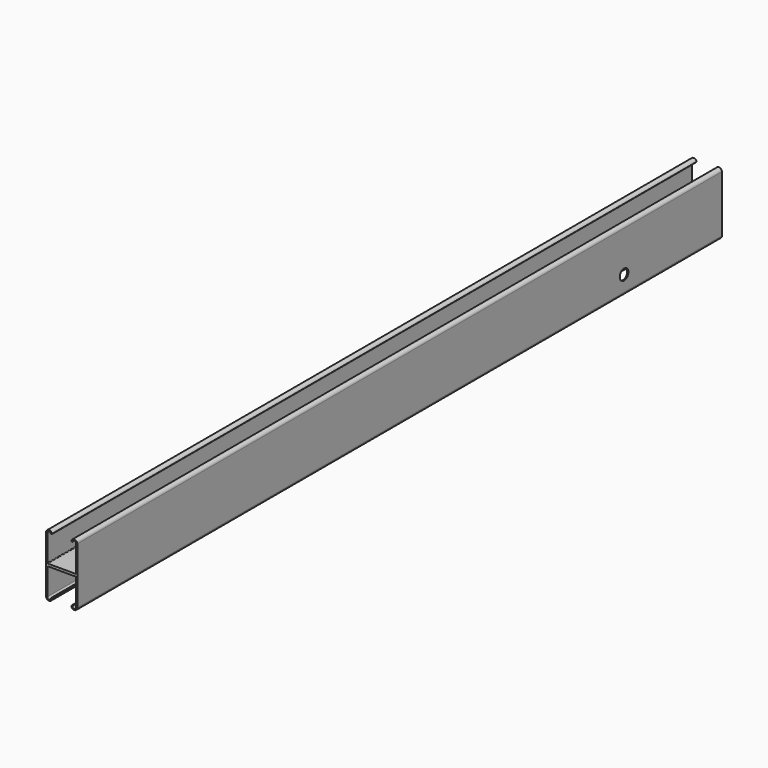
from build123d import *

# Parameters (mm, degrees)
F1_DEPTH = 533.4
F2_R     = 0.79374
F3_R     = 7.14375
F4_DEPTH = 41.276


# Not quite as in the source:
# - a fillet or chamfer is up to 0.001 mm smaller than in the source, because OpenCascade refuses the exact size


with BuildPart() as f1:
    # F0 (on Front) → F1 (new body, symmetric)
    with BuildSketch(Plane.XZ):
        with BuildLine():
            Line((0, 37.30625), (0, 0))
            Line((0, 0), (20.6375, 0))
            Line((20.6375, 0), (20.6375, 1.5875))
            Line((20.6375, 1.5875), (1.5875, 1.5875))
            Line((1.5875, 1.5875), (1.5875, 37.30625))
            ThreePointArc((1.5875, 37.30625), (3.96875, 39.6875), (6.35, 37.30625))
            Line((6.35, 37.30625), (7.9375, 37.30625))
            ThreePointArc((7.9375, 37.30625), (3.96875, 41.275), (0, 37.30625))
        make_face()
        with BuildLine():
            Line((20.6375, 0), (0, 0))
            Line((0, 0), (0, -37.30625))
            ThreePointArc((0, -37.30625), (3.96875, -41.275), (7.9375, -37.30625))
            Line((7.9375, -37.30625), (6.35, -37.30625))
            ThreePointArc((6.35, -37.30625), (3.96875, -39.6875), (1.5875, -37.30625))
            Line((1.5875, -37.30625), (1.5875, -1.5875))
            Line((1.5875, -1.5875), (20.6375, -1.5875))
            Line((20.6375, -1.5875), (20.6375, 0))
        make_face()
        with BuildLine():
            Line((20.6375, 1.5875), (20.6375, 0))
            Line((20.6375, 0), (41.275, 0))
            Line((41.275, 0), (41.275, 37.30625))
            ThreePointArc((41.275, 37.30625), (37.30625, 41.275), (33.3375, 37.30625))
            Line((33.3375, 37.30625), (34.925, 37.30625))
            ThreePointArc((34.925, 37.30625), (37.30625, 39.6875), (39.6875, 37.30625))
            Line((39.6875, 37.30625), (39.6875, 1.5875))
            Line((39.6875, 1.5875), (20.6375, 1.5875))
        make_face()
        with BuildLine():
            Line((41.275, 0), (20.6375, 0))
            Line((20.6375, 0), (20.6375, -1.5875))
            Line((20.6375, -1.5875), (39.6875, -1.5875))
            Line((39.6875, -1.5875), (39.6875, -37.30625))
            ThreePointArc((39.6875, -37.30625), (37.30625, -39.6875), (34.925, -37.30625))
            Line((34.925, -37.30625), (33.3375, -37.30625))
            ThreePointArc((33.3375, -37.30625), (37.30625, -41.275), (41.275, -37.30625))
            Line((41.275, -37.30625), (41.275, 0))
        make_face()
    extrude(amount=F1_DEPTH, both=True)

    # F2 (radius 0.79375 in the source; OpenCascade refuses exactly that, so slightly less here)
    f2_edges = [f1.edges().sort_by_distance(p)[0] for p in [
        (6.35, 0, 37.30625),
        (7.9375, 0, 37.30625),
        (33.3375, 0, 37.30625),
        (34.925, 0, 37.30625),
        (0, 0, 37.30625),
        (41.275, 0, 37.30625),
        (39.6875, 0, 1.5875),
        (1.5875, 0, 1.5875),
    ]]
    fillet(f2_edges, radius=F2_R)

    # F3 (on face) → F4 (cut, through all)
    with BuildSketch(Plane.YZ.offset(41.275)):
        with Locations((371.475, -16.66875)):
            Circle(F3_R)
    extrude(amount=-F4_DEPTH, mode=Mode.SUBTRACT)


solid = f1.part
